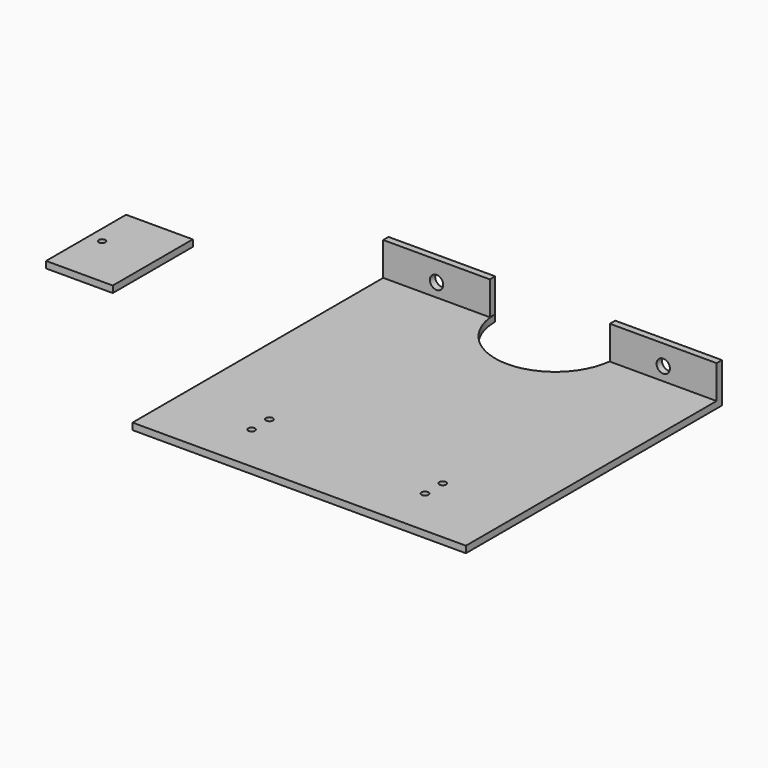
from build123d import *

# Parameters (mm, degrees)
F2_DEPTH = 3.175
F1_W     = 50.8
F1_H     = 19.05
F1_R     = 3.175
F3_DEPTH = 3.175
F5_W     = 31.75
F5_H     = 47.625
F5_R     = 1.5875
F6_DEPTH = 3.175
F7_R     = 1.63195
F8_DEPTH = 39.37


# Not quite as in the source:
# - a feature names something its author has since deleted; it is built from what else it names


with BuildPart() as f2:
    # F0 (on Top) → F2 (new body)
    with BuildSketch(Plane.XY):
        with BuildLine():
            Line((-28.575, 0), (-79.375, 0))
            Line((-79.375, 0), (-79.375, -152.4))
            Line((-79.375, -152.4), (79.375, -152.4))
            Line((79.375, -152.4), (79.375, 0))
            Line((79.375, 0), (28.575, 0))
            ThreePointArc((28.575, 0), (0, -28.575), (-28.575, 0))
        make_face()
    extrude(amount=F2_DEPTH)

    # F1 (on Front) → F3 (join)
    with BuildSketch(Plane.XZ):
        with Locations((53.975, 9.525)):
            Rectangle(F1_W, F1_H)
        with Locations((53.975, 9.525)):
            Circle(F1_R, mode=Mode.SUBTRACT)
        with Locations((-53.975, 9.525)):
            Rectangle(F1_W, F1_H)
        with Locations((-53.975, 9.525)):
            Circle(F1_R, mode=Mode.SUBTRACT)
    extrude(amount=F3_DEPTH)

    # F7 (on Top) → F8 (cut)
    with BuildSketch(Plane.XY):
        with Locations((-41.275, -118.5333333333)):
            Circle(F7_R)
        with Locations((-41.275, -129.1166666667)):
            Circle(F7_R)
        with Locations((41.275, -118.5333333333)):
            Circle(F7_R)
        with Locations((41.275, -129.1166666667)):
            Circle(F7_R)
    extrude(amount=F8_DEPTH, mode=Mode.SUBTRACT)


with BuildPart() as f6:
    # F5 (on Top) → F6 (new body)
    with BuildSketch(Plane.XY):
        with Locations((-169.9210062872, -47.0178964723)):
            Rectangle(F5_W, F5_H)
        with Locations((-179.4460062872, -45.4303964723)):
            Circle(F5_R, mode=Mode.SUBTRACT)
    extrude(amount=F6_DEPTH)


solid = Compound([f2.part, f6.part])
